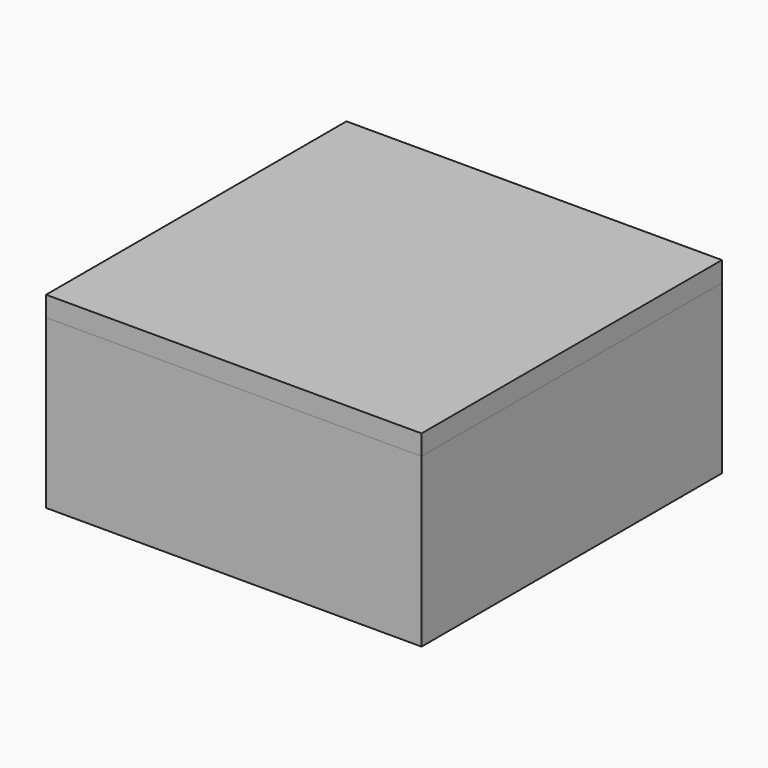
from build123d import *

# Parameters (mm, degrees)
F0_W     = 44.45
F0_H     = 19.84375
F1_DEPTH = 44.45
F2_W     = 44.45
F2_H     = 2.38125
F3_DEPTH = 44.45


# Not quite as in the source:
# - a feature names something its author has since deleted; it is built from what else it names


with BuildPart() as f1:
    # F0 (on Front) → F1 (new body)
    with BuildSketch(Plane.XZ):
        with Locations((22.225, 9.921875)):
            Rectangle(F0_W, F0_H)
    extrude(amount=F1_DEPTH)


with BuildPart() as f3:
    # F2 (on Front) → F3 (new body)
    with BuildSketch(Plane.XZ):
        with Locations((22.225, 21.034375)):
            Rectangle(F2_W, F2_H)
    extrude(amount=F3_DEPTH)


solid = Compound([f1.part, f3.part])
